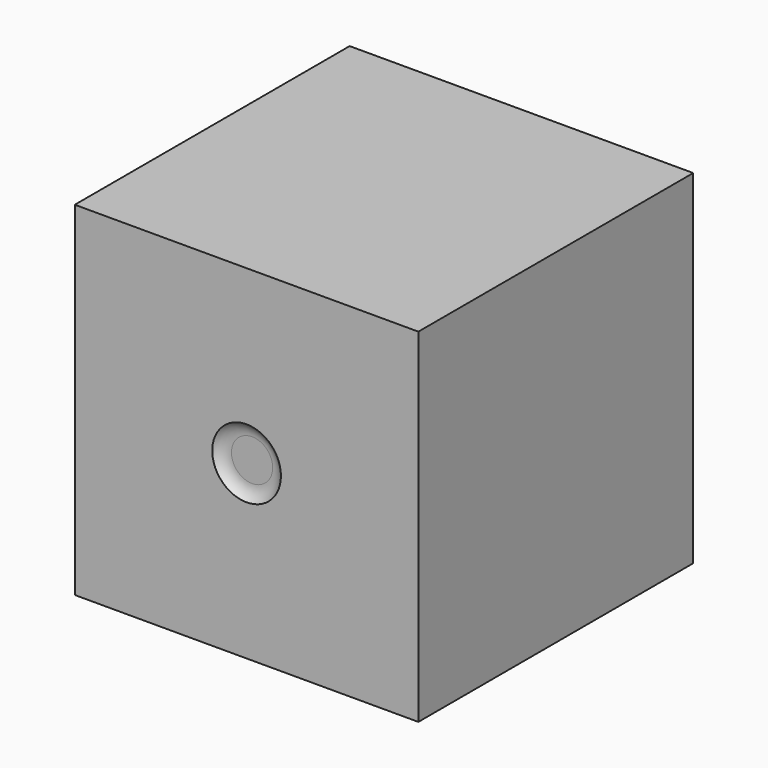
from build123d import *

# Parameters (mm, degrees)
F0_W     = 25.4
F0_H     = 25.4
F1_DEPTH = 25.4
F2_R     = 2.54
F3_DEPTH = 0.508


# Not quite as in the source:
# - a fillet or chamfer that OpenCascade refuses, or shapes differently, is made with other operations: its cross-section is extruded or revolved along the edge and cut away or added


with BuildPart() as f1:
    # F0 (on Front) → F1 (new body)
    with BuildSketch(Plane.XZ):
        Rectangle(F0_W, F0_H)
    extrude(amount=F1_DEPTH)

    # F2 (on face) → F3 (cut)
    with BuildSketch(Plane.XZ.offset(25.4)):
        Circle(F2_R)
    extrude(amount=-F3_DEPTH, mode=Mode.SUBTRACT)

    # F4: fillet of radius 1.27 on 1 edges, made by hand

    # F4_s1 → F4_t2 (revolve)
    with BuildSketch(Plane.XY):
        with BuildLine():
            ThreePointArc((2.54, -25.4), (2.0919612663, -25.0260774674), (1.524, -24.892))
            Line((1.524, -24.892), (2.54, -24.892))
            Line((2.54, -24.892), (2.54, -25.4))
        make_face()
    revolve(axis=Axis((0, -24.892, 0), (0, -1, 0)))


solid = f1.part
